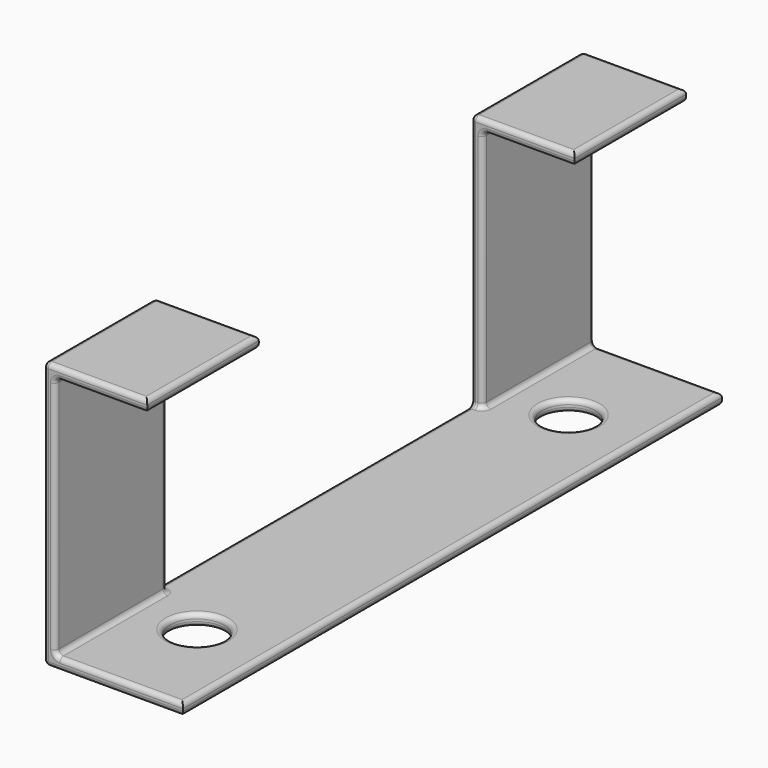
from build123d import *

# Parameters (mm, degrees)
F0_W     = 38.1
F0_H     = 184.15
F0_R     = 7.3152
F0_R_2   = 7.2009
F1_DEPTH = 3.175
F3_W     = 3.175
F3_H     = 38.1
F4_DEPTH = 69.85
F6_W     = 38.1
F6_H     = 3.175
F7_DEPTH = 25.4
F8_R     = 1.27


with BuildPart() as f1:
    # F0 (on Top) → F1 (new body)
    with BuildSketch(Plane.XY):
        Rectangle(F0_W, F0_H)
        with Locations((0, -63.5)):
            Circle(F0_R, mode=Mode.SUBTRACT)
        with Locations((0, 63.5)):
            Circle(F0_R_2, mode=Mode.SUBTRACT)
    extrude(amount=F1_DEPTH)

    # F3 (on offset) → F4 (join)
    with BuildSketch(Plane.XY.offset(3.175)):
        with Locations((-17.4625, 73.025)):
            Rectangle(F3_W, F3_H)
        with Locations((-17.4625, -73.025)):
            Rectangle(F3_W, F3_H)
    extrude(amount=F4_DEPTH)

    # F6 (on offset) → F7 (join)
    with BuildSketch(Plane.YZ.offset(-16.129)):
        with Locations((-73.025, 71.4375)):
            Rectangle(F6_W, F6_H)
        with Locations((73.025, 71.4375)):
            Rectangle(F6_W, F6_H)
    extrude(amount=F7_DEPTH)

    # F8
    f8_edges = [f1.edges().sort_by_distance(p)[0] for p in [
        (-15.875, 73.025, 3.175),
        (-15.875, 92.075, 36.5125),
        (-15.875, 73.025, 69.85),
        (-15.875, 53.975, 36.5125),
        (-19.05, 0, 0),
        (0, -92.075, 0),
        (19.05, 0, 0),
        (0, 92.075, 0),
        (-7.3152, -63.5, 0),
        (-7.2009, 63.5, 0),
        (-3.302, 92.075, 69.85),
        (9.271, 73.025, 69.85),
        (-3.302, 53.975, 69.85),
        (-15.875, -73.025, 69.85),
        (-3.302, -53.975, 69.85),
        (9.271, -73.025, 69.85),
        (-3.302, -92.075, 69.85),
        (-4.8895, -92.075, 73.025),
        (9.271, -73.025, 73.025),
        (-4.8895, -53.975, 73.025),
        (-19.05, -73.025, 73.025),
        (-4.8895, 53.975, 73.025),
        (9.271, 73.025, 73.025),
        (-4.8895, 92.075, 73.025),
        (-19.05, 73.025, 73.025),
        (-17.4625, 53.975, 3.175),
        (1.5875, 92.075, 3.175),
        (19.05, 0, 3.175),
        (1.5875, -92.075, 3.175),
        (-15.875, -73.025, 3.175),
        (-17.4625, -53.975, 3.175),
        (-19.05, 0, 3.175),
        (-7.3152, -63.5, 3.175),
        (-7.2009, 63.5, 3.175),
        (-19.05, -92.075, 36.5125),
        (-19.05, -53.975, 38.1),
        (-19.05, 92.075, 36.5125),
        (-19.05, 53.975, 38.1),
        (-15.875, -92.075, 36.5125),
        (-15.875, -53.975, 36.5125),
    ]]
    fillet(f8_edges, radius=F8_R)


solid = f1.part
